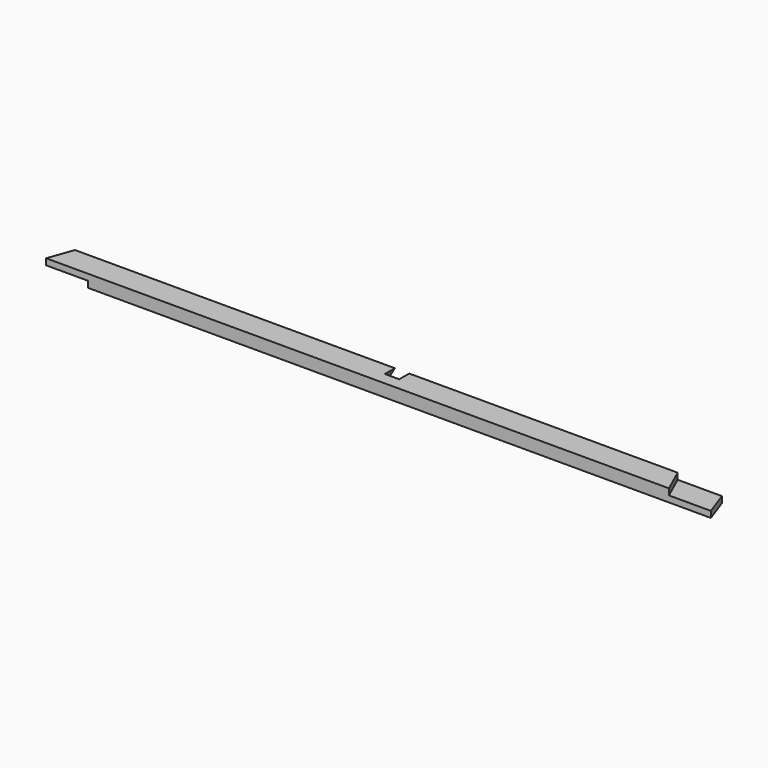
from build123d import *

# Parameters (mm, degrees)
F0_W      = 1016
F0_H      = 19.05
F1_DEPTH  = 38.1
F3_DEPTH  = 50.8
F5_DEPTH  = 76.2
F7_DEPTH  = 60.325
F9_DEPTH  = 9.525
F11_DEPTH = 60.325
F13_DEPTH = 19.05
F15_DEPTH = 9.525


with BuildPart() as f1:
    # F0 (on Front) → F1 (new body)
    with BuildSketch(Plane.XZ):
        with Locations((-508, 9.525)):
            Rectangle(F0_W, F0_H)
    extrude(amount=F1_DEPTH)

    # F2 (on face) → F3 (cut)
    with BuildSketch(Plane.XY.offset(19.05)):
        Polygon((-1016, 0), (-1016, -38.1), (-1002.3770791998, 0), align=None)
    extrude(amount=-F3_DEPTH, mode=Mode.SUBTRACT)

    # F4 (on face) → F5 (cut)
    with BuildSketch(Plane.XY.offset(19.05)):
        Polygon((-13.6229208002, 0), (0, -38.1), (0, 0), align=None)
    extrude(amount=-F5_DEPTH, mode=Mode.SUBTRACT)

    # F6 (on face) → F7 (cut)
    with BuildSketch(Plane(origin=(-888.7527181239, 317.7797346454, 0), x_dir=(-0.3366822055, -0.941618337, 0), z_dir=(-0.941618337, 0.3366822055, 0))):
        Polygon((252.7767419815, 9.525), (258.7343550339, 0), (377.9447794005, 0), (377.9447794005, 9.525), align=None)
    extrude(amount=-F7_DEPTH, mode=Mode.SUBTRACT)

    # F8 (on face) → F9 (cut)
    with BuildSketch(Plane(origin=(0, 0, 0), x_dir=(1, 0, 0), z_dir=(0, 0, -1))):
        Polygon((-951.9347650406, 38.1), (-951.9347650406, 0), (-934.7637907817, 0), align=None)
    extrude(amount=-F9_DEPTH, mode=Mode.SUBTRACT)

    # F10 (on face) → F11 (cut)
    with BuildSketch(Plane(origin=(-12.0786958733, -4.3188219751, 0), x_dir=(-0.3366822055, 0.941618337, 0), z_dir=(0.941618337, 0.3366822055, 0))):
        Polygon((-35.8756586385, 19.05), (-35.8756586385, 9.525), (45.2719508199, 9.525), (45.6329248846, 19.05), align=None)
    extrude(amount=-F11_DEPTH, mode=Mode.SUBTRACT)

    # F12 (on face) → F13 (cut)
    with BuildSketch(Plane(origin=(0, 0, 0), x_dir=(-1, 0, 0), z_dir=(0, 1, 0))):
        Polygon((524.497778814, 0), (513.499256186, 19.05), (491.502221186, 19.05), (502.500743814, 0), align=None)
    extrude(amount=-F13_DEPTH, mode=Mode.SUBTRACT)

    # F14 (on face) → F15 (cut)
    with BuildSketch(Plane.XY.offset(19.05)):
        Polygon((-64.0652349594, 0), (-81.2362092183, 0), (-64.0652349594, -38.1), align=None)
    extrude(amount=-F15_DEPTH, mode=Mode.SUBTRACT)


solid = f1.part
